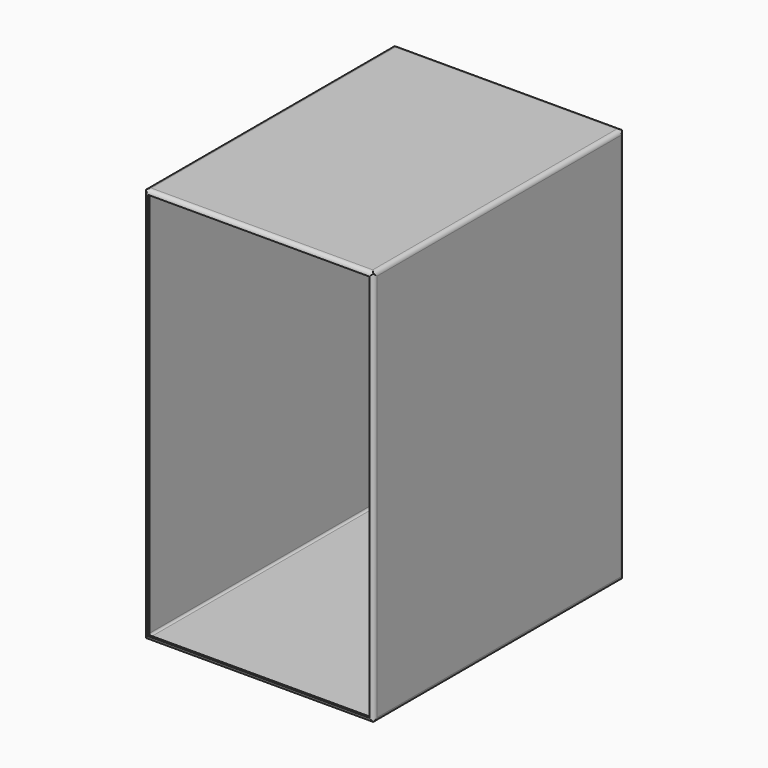
from build123d import *

# Parameters (mm, degrees)
F0_W        = 279.4
F0_H        = 482.6
F1_DEPTH    = 381
F2_R        = 5.08
F3_T1_DEPTH = 401.32
F3_T3_DEPTH = 508
F4_T1_DEPTH = 299.72
F4_T3_DEPTH = 508
F5_T1_DEPTH = 396.24
F6_T        = -2.54


# Not quite as in the source:
# - a fillet or chamfer that OpenCascade refuses, or shapes differently, is made with other operations: its cross-section is extruded or revolved along the edge and cut away or added
# - a shell that OpenCascade refuses in one call is made with other operations: the cavity is built on its own and cut out


with BuildPart() as f1:
    # F0 (on Front) → F1 (new body)
    with BuildSketch(Plane.XZ):
        Rectangle(F0_W, F0_H)
    extrude(amount=F1_DEPTH)

    # F2
    f2_edges = [f1.edges().sort_by_distance(p)[0] for p in [
        (-139.7, -381, 0),
        (0, -381, -241.3),
        (139.7, -381, 0),
        (0, -381, 241.3),
    ]]
    fillet(f2_edges, radius=F2_R)

    # F3: fillet of radius 5.08 on 4 edges, made by hand

    # F3_s2 → F3_t1 (cut)
    with BuildSketch(Plane.XZ.offset(-12.7)):
        with BuildLine():
            ThreePointArc((-139.7, 236.22), (-138.2121024484, 239.8121024484), (-134.62, 241.3))
            Line((-134.62, 241.3), (-139.7, 241.3))
            Line((-139.7, 241.3), (-139.7, 236.22))
        make_face()
        with BuildLine():
            ThreePointArc((-139.7, -236.22), (-138.2121024484, -239.8121024484), (-134.62, -241.3))
            Line((-134.62, -241.3), (-139.7, -241.3))
            Line((-139.7, -241.3), (-139.7, -236.22))
        make_face()
    extrude(amount=F3_T1_DEPTH, mode=Mode.SUBTRACT)

    # F3_s4 → F3_t3 (cut)
    with BuildSketch(Plane.XY.offset(-254)):
        with BuildLine():
            ThreePointArc((-139.7, -5.08), (-138.2121024484, -1.4878975516), (-134.62, 0))
            Line((-134.62, 0), (-139.7, 0))
            Line((-139.7, 0), (-139.7, -5.08))
        make_face()
    extrude(amount=F3_T3_DEPTH, mode=Mode.SUBTRACT)

    # F4: fillet of radius 5.08 on 4 edges, made by hand

    # F4_s2 → F4_t1 (cut)
    with BuildSketch(Plane.YZ.offset(-147.32)):
        with BuildLine():
            ThreePointArc((0, 236.22), (-1.4878975516, 239.8121024484), (-5.08, 241.3))
            Line((-5.08, 241.3), (0, 241.3))
            Line((0, 241.3), (0, 236.22))
        make_face()
        with BuildLine():
            ThreePointArc((0, -236.22), (-1.4878975516, -239.8121024484), (-5.08, -241.3))
            Line((-5.08, -241.3), (0, -241.3))
            Line((0, -241.3), (0, -236.22))
        make_face()
    extrude(amount=F4_T1_DEPTH, mode=Mode.SUBTRACT)

    # F4_s4 → F4_t3 (cut)
    with BuildSketch(Plane.XY.offset(-254)):
        with BuildLine():
            ThreePointArc((134.62, 0), (138.2121024484, -1.4878975516), (139.7, -5.08))
            Line((139.7, -5.08), (139.7, 0))
            Line((139.7, 0), (134.62, 0))
        make_face()
    extrude(amount=F4_T3_DEPTH, mode=Mode.SUBTRACT)

    # F5: fillet of radius 5.08 on 4 edges, made by hand

    # F5_s2 → F5_t1 (cut)
    with BuildSketch(Plane.XZ.offset(-7.62)):
        with BuildLine():
            ThreePointArc((134.62, 241.3), (138.2121024484, 239.8121024484), (139.7, 236.22))
            Line((139.7, 236.22), (139.7, 241.3))
            Line((139.7, 241.3), (134.62, 241.3))
        make_face()
        with BuildLine():
            ThreePointArc((134.62, -241.3), (138.2121024484, -239.8121024484), (139.7, -236.22))
            Line((139.7, -236.22), (139.7, -241.3))
            Line((139.7, -241.3), (134.62, -241.3))
        make_face()
    extrude(amount=F5_T1_DEPTH, mode=Mode.SUBTRACT)

    # F6: a shell. OpenCascade refuses it in one call, so the cavity is built on its own and cut out:
    # the body offset inwards by the wall thickness, plus a prism from it out through each open face.
    f6_core = offset(f1.part, amount=F6_T, mode=Mode.PRIVATE)
    f6_exits = [f6_core.faces().sort_by_distance(p)[0] for p in [
        (0, -378.46, 0),
    ]]
    add(f6_core, mode=Mode.SUBTRACT)
    extrude(f6_exits, amount=-F6_T, mode=Mode.SUBTRACT)


solid = f1.part
